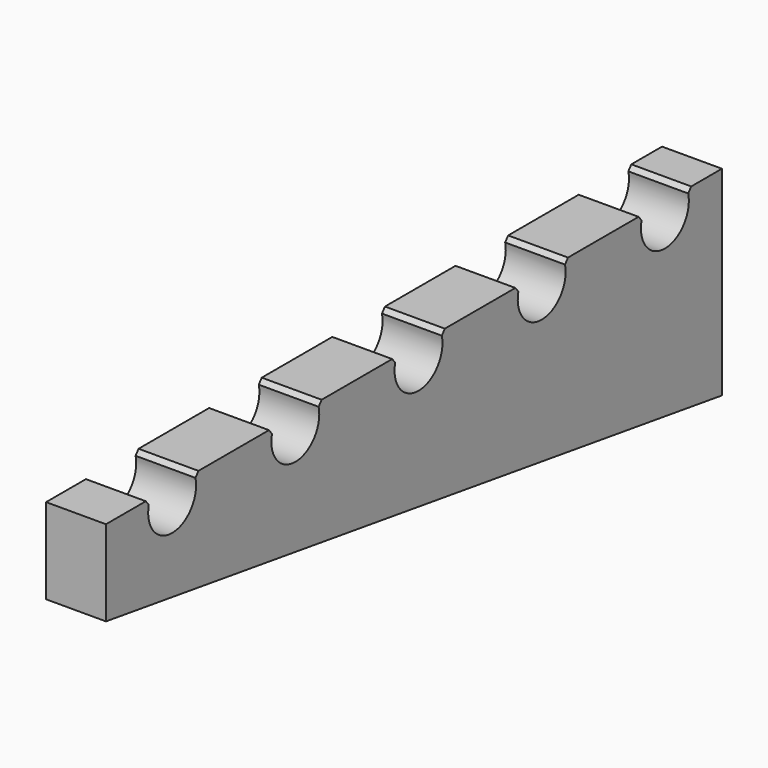
from build123d import *

# Parameters (mm, degrees)
F1_DEPTH    = 21
F2_R        = 10.5
F3_DEPTH    = 25
F4_T1_DEPTH = 30.3938312155


# Not quite as in the source:
# - a fillet or chamfer that OpenCascade refuses, or shapes differently, is made with other operations: its cross-section is extruded or revolved along the edge and cut away or added


with BuildPart() as f1:
    # F0 (on Right) → F1 (new body)
    with BuildSketch(Plane.YZ):
        Polygon((-135, -5), (135, -45), (135, 25), (-135, 25), align=None)
    extrude(amount=F1_DEPTH)

    # F2 (on face) → F3 (cut)
    with BuildSketch(Plane.YZ.offset(21)):
        with Locations((110, 21)):
            Circle(F2_R)
        with Locations((56, 21)):
            Circle(F2_R)
        with Locations((2, 21)):
            Circle(F2_R)
        with Locations((-52, 21)):
            Circle(F2_R)
        with Locations((-106, 21)):
            Circle(F2_R)
    extrude(amount=-F3_DEPTH, mode=Mode.SUBTRACT)

    # F4: chamfer of 2 on 10 edges, made by hand

    # F4_s2 → F4_t1 (cut)
    with BuildSketch(Plane.YZ.offset(-4.6969156077)):
        with BuildLine():
            Line((-117.5859668407, 25.062603733), (-116.1815447498, 23.2973611197))
            Line((-116.1815447498, 23.2973611197), (-116.1425681704, 23.2883707774))
            ThreePointArc((-116.1425681704, 23.2883707774), (-115.9721143456, 24.157298763), (-115.6712601331, 24.9847619048))
            Line((-115.6712601331, 24.9847619048), (-115.7082439195, 25.04))
            ThreePointArc((-115.7082439195, 25.04), (-116.6471053801, 25.04), (-117.5859668407, 25.102603733))
            Line((-117.5859668407, 25.102603733), (-117.5859668407, 25.062603733))
        make_face()
        with BuildLine():
            Line((-95.8184552502, 23.2973611197), (-94.4140331593, 25.062603733))
            Line((-94.4140331593, 25.062603733), (-94.4140331593, 25.102603733))
            ThreePointArc((-94.4140331593, 25.102603733), (-95.3528946199, 25.04), (-96.2917560805, 25.04))
            Line((-96.2917560805, 25.04), (-96.3287398669, 24.9847619048))
            ThreePointArc((-96.3287398669, 24.9847619048), (-96.0278856544, 24.157298763), (-95.8574318296, 23.2883707774))
            Line((-95.8574318296, 23.2883707774), (-95.8184552502, 23.2973611197))
        make_face()
        with BuildLine():
            Line((-63.5859668407, 25.062603733), (-62.1815447498, 23.2973611197))
            Line((-62.1815447498, 23.2973611197), (-62.1425681704, 23.2883707774))
            ThreePointArc((-62.1425681704, 23.2883707774), (-61.9721143456, 24.157298763), (-61.6712601331, 24.9847619048))
            Line((-61.6712601331, 24.9847619048), (-61.7082439195, 25.04))
            ThreePointArc((-61.7082439195, 25.04), (-62.6471053801, 25.04), (-63.5859668407, 25.102603733))
            Line((-63.5859668407, 25.102603733), (-63.5859668407, 25.062603733))
        make_face()
        with BuildLine():
            Line((-41.8184552502, 23.2973611197), (-40.4140331593, 25.062603733))
            Line((-40.4140331593, 25.062603733), (-40.4140331593, 25.102603733))
            ThreePointArc((-40.4140331593, 25.102603733), (-41.3528946199, 25.04), (-42.2917560805, 25.04))
            Line((-42.2917560805, 25.04), (-42.3287398669, 24.9847619048))
            ThreePointArc((-42.3287398669, 24.9847619048), (-42.0278856544, 24.157298763), (-41.8574318296, 23.2883707774))
            Line((-41.8574318296, 23.2883707774), (-41.8184552502, 23.2973611197))
        make_face()
        with BuildLine():
            Line((-9.5859668407, 25.062603733), (-8.1815447498, 23.2973611197))
            Line((-8.1815447498, 23.2973611197), (-8.1425681704, 23.2883707774))
            ThreePointArc((-8.1425681704, 23.2883707774), (-7.9721143456, 24.157298763), (-7.6712601331, 24.9847619048))
            Line((-7.6712601331, 24.9847619048), (-7.7082439195, 25.04))
            ThreePointArc((-7.7082439195, 25.04), (-8.6471053801, 25.04), (-9.5859668407, 25.102603733))
            Line((-9.5859668407, 25.102603733), (-9.5859668407, 25.062603733))
        make_face()
        with BuildLine():
            Line((12.1815447498, 23.2973611197), (13.5859668407, 25.062603733))
            Line((13.5859668407, 25.062603733), (13.5859668407, 25.102603733))
            ThreePointArc((13.5859668407, 25.102603733), (12.6471053801, 25.04), (11.7082439195, 25.04))
            Line((11.7082439195, 25.04), (11.6712601331, 24.9847619048))
            ThreePointArc((11.6712601331, 24.9847619048), (11.9721143456, 24.157298763), (12.1425681704, 23.2883707774))
            Line((12.1425681704, 23.2883707774), (12.1815447498, 23.2973611197))
        make_face()
        with BuildLine():
            Line((44.4140331593, 25.062603733), (45.8184552502, 23.2973611197))
            Line((45.8184552502, 23.2973611197), (45.8574318296, 23.2883707774))
            ThreePointArc((45.8574318296, 23.2883707774), (46.0278856544, 24.157298763), (46.3287398669, 24.9847619048))
            Line((46.3287398669, 24.9847619048), (46.2917560805, 25.04))
            ThreePointArc((46.2917560805, 25.04), (45.3528946199, 25.04), (44.4140331593, 25.102603733))
            Line((44.4140331593, 25.102603733), (44.4140331593, 25.062603733))
        make_face()
        with BuildLine():
            Line((66.1815447498, 23.2973611197), (67.5859668407, 25.062603733))
            Line((67.5859668407, 25.062603733), (67.5859668407, 25.102603733))
            ThreePointArc((67.5859668407, 25.102603733), (66.6471053801, 25.04), (65.7082439195, 25.04))
            Line((65.7082439195, 25.04), (65.6712601331, 24.9847619048))
            ThreePointArc((65.6712601331, 24.9847619048), (65.9721143456, 24.157298763), (66.1425681704, 23.2883707774))
            Line((66.1425681704, 23.2883707774), (66.1815447498, 23.2973611197))
        make_face()
        with BuildLine():
            Line((98.4140331593, 25.062603733), (99.8184552502, 23.2973611197))
            Line((99.8184552502, 23.2973611197), (99.8574318296, 23.2883707774))
            ThreePointArc((99.8574318296, 23.2883707774), (100.0278856544, 24.157298763), (100.3287398669, 24.9847619048))
            Line((100.3287398669, 24.9847619048), (100.2917560805, 25.04))
            ThreePointArc((100.2917560805, 25.04), (99.3528946199, 25.04), (98.4140331593, 25.102603733))
            Line((98.4140331593, 25.102603733), (98.4140331593, 25.062603733))
        make_face()
        with BuildLine():
            Line((120.1815447498, 23.2973611197), (121.5859668407, 25.062603733))
            Line((121.5859668407, 25.062603733), (121.5859668407, 25.102603733))
            ThreePointArc((121.5859668407, 25.102603733), (120.6471053801, 25.04), (119.7082439195, 25.04))
            Line((119.7082439195, 25.04), (119.6712601331, 24.9847619048))
            ThreePointArc((119.6712601331, 24.9847619048), (119.9721143456, 24.157298763), (120.1425681704, 23.2883707774))
            Line((120.1425681704, 23.2883707774), (120.1815447498, 23.2973611197))
        make_face()
    extrude(amount=F4_T1_DEPTH, mode=Mode.SUBTRACT)


solid = f1.part
